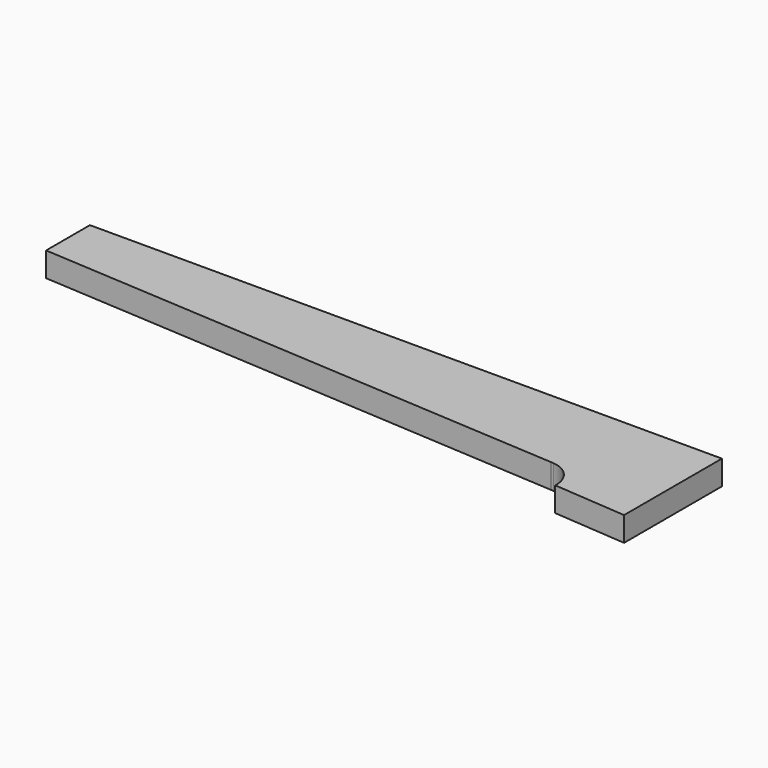
from build123d import *

# Parameters (mm, degrees)
F2_DEPTH    = 3
F3_T1_DEPTH = 3.3473896723


# Not quite as in the source:
# - a fillet or chamfer that OpenCascade refuses, or shapes differently, is made with other operations: its cross-section is extruded or revolved along the edge and cut away or added


with BuildPart() as f2:
    # F1 (on face) → F2 (new body)
    with BuildSketch(Plane.XY):
        with BuildLine():
            Line((23.5, -3.5), (20.4928553643, -3.3120534603))
            ThreePointArc((20.4928553643, -3.3120534603), (22.5915627309, -4.3550902955), (23.5, -6.5154699331))
            Line((23.5, -6.5154699331), (23.5, -3.5))
        make_face()
        with BuildLine():
            Line((-32.5, 7.5), (-32.5, 0))
            Line((-32.5, 0), (20.2037399466, -3.2939837467))
            ThreePointArc((20.2037399466, -3.2939837467), (20.3484922252, -3.2999054879), (20.4928553643, -3.3120534603))
            Line((20.4928553643, -3.3120534603), (23.5, -3.5))
            Line((23.5, -3.5), (23.5, -6.5154699331))
            ThreePointArc((23.5, -6.5154699331), (23.5030092301, -6.6577349666), (23.5, -6.8))
            Line((23.5, -6.8), (32.5, -7.5))
            Line((32.5, -7.5), (32.5, 7.5))
            Line((32.5, 7.5), (-32.5, 7.5))
        make_face()
        Polygon((-45, 0.78125), (-32.5, 0), (-32.5, 7.5), (-45, 7.5), align=None)
    extrude(amount=F2_DEPTH)

    # F3: fillet of radius 4 on 1 edges, made by hand

    # F3_s2 → F3_t1 (cut)
    with BuildSketch(Plane.XY.offset(-0.1736948361)):
        with BuildLine():
            ThreePointArc((20.134397315, -3.2896498322), (20.1925204005, -3.2928581253), (20.2506840199, -3.2952202421))
            ThreePointArc((20.2506840199, -3.2952202421), (20.2272141407, -3.2945200871), (20.2037399466, -3.2939837467))
            Line((20.2037399466, -3.2939837467), (20.134397315, -3.2896498322))
        make_face()
    extrude(amount=F3_T1_DEPTH, mode=Mode.SUBTRACT)


solid = f2.part
